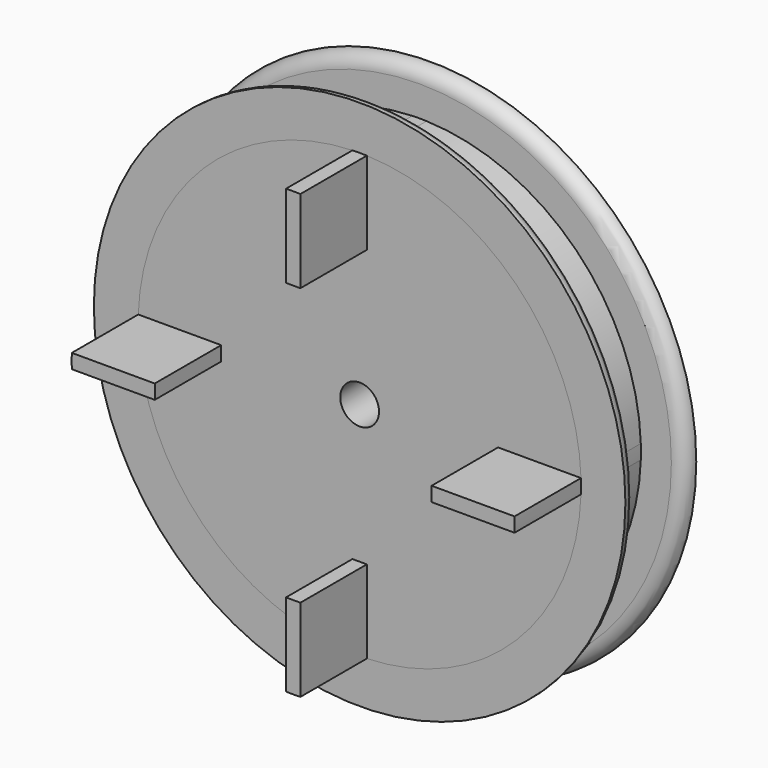
from build123d import *

# Parameters (mm, degrees)
F0_R     = 24
F0_R_2   = 1.75
F1_DEPTH = 8
F2_DEPTH = 6.75
F3_DEPTH = 1.25
F4_R     = 1.24999
F4_2_R   = 1.24999
F5_DEPTH = 7.5


# Not quite as in the source:
# - a fillet or chamfer is up to 0.001 mm smaller than in the source, because OpenCascade refuses the exact size
# - after a boolean that leaves OpenCascade's solid faulty, fix() repairs it


with BuildPart() as f1:
    # F0 (on Front) → F1 (new body)
    with BuildSketch(Plane.XZ):
        Circle(F0_R)
        with BuildLine():
            ThreePointArc((19.9894375, 0.649914174), (19.9973592007, 0.325), (20, 0))
            ThreePointArc((20, 0), (19.9973592007, -0.325), (19.9894375, -0.649914174))
            ThreePointArc((19.9894375, -0.649914174), (14.1421356237, -14.1421356237), (0.649914174, -19.9894375))
            ThreePointArc((0.649914174, -19.9894375), (0, -20), (-0.649914174, -19.9894375))
            ThreePointArc((-0.649914174, -19.9894375), (-14.1421356237, -14.1421356237), (-19.9894375, -0.649914174))
            ThreePointArc((-19.9894375, -0.649914174), (-20, 0), (-19.9894375, 0.649914174))
            ThreePointArc((-19.9894375, 0.649914174), (-14.1421356237, 14.1421356237), (-0.649914174, 19.9894375))
            ThreePointArc((-0.649914174, 19.9894375), (0, 20), (0.649914174, 19.9894375))
            ThreePointArc((0.649914174, 19.9894375), (14.1421356237, 14.1421356237), (19.9894375, 0.649914174))
        make_face(mode=Mode.SUBTRACT)
        with BuildLine():
            Line((12.5, 0.649914174), (19.9894375, 0.649914174))
            ThreePointArc((19.9894375, 0.649914174), (14.1421356237, 14.1421356237), (0.649914174, 19.9894375))
            Line((0.649914174, 19.9894375), (0.649914174, 12.5))
            Line((0.649914174, 12.5), (-0.649914174, 12.5))
            Line((-0.649914174, 12.5), (-0.649914174, 19.9894375))
            ThreePointArc((-0.649914174, 19.9894375), (-14.1421356237, 14.1421356237), (-19.9894375, 0.649914174))
            Line((-19.9894375, 0.649914174), (-12.5, 0.649914174))
            Line((-12.5, 0.649914174), (-12.5, -0.649914174))
            Line((-12.5, -0.649914174), (-19.9894375, -0.649914174))
            ThreePointArc((-19.9894375, -0.649914174), (-14.1421356237, -14.1421356237), (-0.649914174, -19.9894375))
            Line((-0.649914174, -19.9894375), (-0.649914174, -12.5))
            Line((-0.649914174, -12.5), (0.649914174, -12.5))
            Line((0.649914174, -12.5), (0.649914174, -19.9894375))
            ThreePointArc((0.649914174, -19.9894375), (14.1421356237, -14.1421356237), (19.9894375, -0.649914174))
            Line((19.9894375, -0.649914174), (12.5, -0.649914174))
            Line((12.5, -0.649914174), (12.5, 0.649914174))
        make_face()
        Circle(F0_R_2, mode=Mode.SUBTRACT)
        with BuildLine():
            Line((0.649914174, 12.5), (0.649914174, 19.9894375))
            ThreePointArc((0.649914174, 19.9894375), (0, 20), (-0.649914174, 19.9894375))
            Line((-0.649914174, 19.9894375), (-0.649914174, 12.5))
            Line((-0.649914174, 12.5), (0.649914174, 12.5))
        make_face()
        with BuildLine():
            ThreePointArc((19.9894375, -0.649914174), (19.9973592007, -0.325), (20, 0))
            ThreePointArc((20, 0), (19.9973592007, 0.325), (19.9894375, 0.649914174))
            Line((19.9894375, 0.649914174), (12.5, 0.649914174))
            Line((12.5, 0.649914174), (12.5, -0.649914174))
            Line((12.5, -0.649914174), (19.9894375, -0.649914174))
        make_face()
        with BuildLine():
            Line((-12.5, 0.649914174), (-19.9894375, 0.649914174))
            ThreePointArc((-19.9894375, 0.649914174), (-20, 0), (-19.9894375, -0.649914174))
            Line((-19.9894375, -0.649914174), (-12.5, -0.649914174))
            Line((-12.5, -0.649914174), (-12.5, 0.649914174))
        make_face()
        with BuildLine():
            ThreePointArc((-0.649914174, -19.9894375), (0, -20), (0.649914174, -19.9894375))
            Line((0.649914174, -19.9894375), (0.649914174, -12.5))
            Line((0.649914174, -12.5), (-0.649914174, -12.5))
            Line((-0.649914174, -12.5), (-0.649914174, -19.9894375))
        make_face()
    extrude(amount=-F1_DEPTH)

    # F0 (on Front) → F2 (cut)
    with BuildSketch(Plane.XZ):
        Circle(F0_R)
        with BuildLine():
            ThreePointArc((19.9894375, 0.649914174), (19.9973592007, 0.325), (20, 0))
            ThreePointArc((20, 0), (19.9973592007, -0.325), (19.9894375, -0.649914174))
            ThreePointArc((19.9894375, -0.649914174), (14.1421356237, -14.1421356237), (0.649914174, -19.9894375))
            ThreePointArc((0.649914174, -19.9894375), (0, -20), (-0.649914174, -19.9894375))
            ThreePointArc((-0.649914174, -19.9894375), (-14.1421356237, -14.1421356237), (-19.9894375, -0.649914174))
            ThreePointArc((-19.9894375, -0.649914174), (-20, 0), (-19.9894375, 0.649914174))
            ThreePointArc((-19.9894375, 0.649914174), (-14.1421356237, 14.1421356237), (-0.649914174, 19.9894375))
            ThreePointArc((-0.649914174, 19.9894375), (0, 20), (0.649914174, 19.9894375))
            ThreePointArc((0.649914174, 19.9894375), (14.1421356237, 14.1421356237), (19.9894375, 0.649914174))
        make_face(mode=Mode.SUBTRACT)
    extrude(amount=-F2_DEPTH, mode=Mode.SUBTRACT)

    # F4 (radius 1.25 in the source; OpenCascade refuses exactly that, so slightly less here)
    f4_edges = [f1.edges().sort_by_distance(p)[0] for p in [
        (-24, 6.75, 0),
    ]]
    fillet(f4_edges, radius=F4_R)

    # F0 (on Front) → F5 (join)
    with BuildSketch(Plane.XZ):
        with BuildLine():
            Line((0.649914174, 12.5), (0.649914174, 19.9894375))
            ThreePointArc((0.649914174, 19.9894375), (0, 20), (-0.649914174, 19.9894375))
            Line((-0.649914174, 19.9894375), (-0.649914174, 12.5))
            Line((-0.649914174, 12.5), (0.649914174, 12.5))
        make_face()
        with BuildLine():
            Line((-12.5, 0.649914174), (-19.9894375, 0.649914174))
            ThreePointArc((-19.9894375, 0.649914174), (-20, 0), (-19.9894375, -0.649914174))
            Line((-19.9894375, -0.649914174), (-12.5, -0.649914174))
            Line((-12.5, -0.649914174), (-12.5, 0.649914174))
        make_face()
        with BuildLine():
            ThreePointArc((19.9894375, -0.649914174), (19.9973592007, -0.325), (20, 0))
            ThreePointArc((20, 0), (19.9973592007, 0.325), (19.9894375, 0.649914174))
            Line((19.9894375, 0.649914174), (12.5, 0.649914174))
            Line((12.5, 0.649914174), (12.5, -0.649914174))
            Line((12.5, -0.649914174), (19.9894375, -0.649914174))
        make_face()
        with BuildLine():
            ThreePointArc((-0.649914174, -19.9894375), (0, -20), (0.649914174, -19.9894375))
            Line((0.649914174, -19.9894375), (0.649914174, -12.5))
            Line((0.649914174, -12.5), (-0.649914174, -12.5))
            Line((-0.649914174, -12.5), (-0.649914174, -19.9894375))
        make_face()
    extrude(amount=F5_DEPTH)

    add(f1.part.fix(), mode=Mode.REPLACE)


with BuildPart() as f3:
    # F0 (on Front) → F3 (new body)
    with BuildSketch(Plane.XZ):
        Circle(F0_R)
        with BuildLine():
            ThreePointArc((19.9894375, 0.649914174), (19.9973592007, 0.325), (20, 0))
            ThreePointArc((20, 0), (19.9973592007, -0.325), (19.9894375, -0.649914174))
            ThreePointArc((19.9894375, -0.649914174), (14.1421356237, -14.1421356237), (0.649914174, -19.9894375))
            ThreePointArc((0.649914174, -19.9894375), (0, -20), (-0.649914174, -19.9894375))
            ThreePointArc((-0.649914174, -19.9894375), (-14.1421356237, -14.1421356237), (-19.9894375, -0.649914174))
            ThreePointArc((-19.9894375, -0.649914174), (-20, 0), (-19.9894375, 0.649914174))
            ThreePointArc((-19.9894375, 0.649914174), (-14.1421356237, 14.1421356237), (-0.649914174, 19.9894375))
            ThreePointArc((-0.649914174, 19.9894375), (0, 20), (0.649914174, 19.9894375))
            ThreePointArc((0.649914174, 19.9894375), (14.1421356237, 14.1421356237), (19.9894375, 0.649914174))
        make_face(mode=Mode.SUBTRACT)
    extrude(amount=-F3_DEPTH)

    # F4#2 (radius 1.25 in the source; OpenCascade refuses exactly that, so slightly less here)
    f4_2_edges = [f3.edges().sort_by_distance(p)[0] for p in [
        (-24, 1.25, 0),
    ]]
    fillet(f4_2_edges, radius=F4_2_R)


solid = Compound([f1.part, f3.part])
